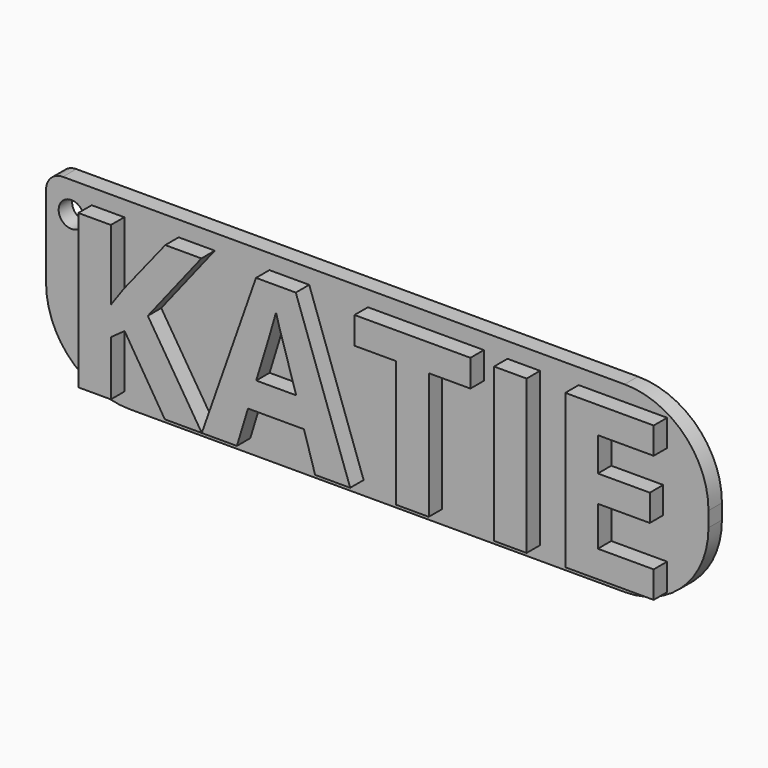
from build123d import *

# Parameters (mm, degrees)
F0_TEXT_SIZE = 32.5522437278
F2_DEPTH     = 5.08
F1_W         = 100.2589799464
F1_H         = 27.6808142662
F3_DEPTH     = 2.54
F4_R         = 12.7
F5_R         = 2.54
F6_R         = 1.9295612823
F7_DEPTH     = 2.54


# Not quite as in the source:
# - Text() gives the source's letters only with a copy of the font that has no kerning and outlines rounded to 1/6400 em; it was checked with that copy


with BuildPart() as f2:
    # F0 (on Front) → F2 (new body)
    with BuildSketch(Plane.XZ):
        with Locations((-40.1719734073, 18.204908818)):
            Text('KATIE', F0_TEXT_SIZE, font='Open Sans', font_style=FontStyle.BOLD, text_align=(TextAlign.LEFT, TextAlign.BOTTOM))
    extrude(amount=F2_DEPTH)


with BuildPart() as f3:
    # F1 (on face) → F3 (new body)
    with BuildSketch(Plane.XZ):
        with Locations((5.9745330364, 29.9661830068)):
            Rectangle(F1_W, F1_H)
    extrude(amount=F3_DEPTH)

    # F4
    f4_edges = [f3.edges().sort_by_distance(p)[0] for p in [
        (-44.154957, -1.27, 16.125776),
        (56.104023, -1.27, 43.80659),
        (56.104023, -1.27, 16.125776),
    ]]
    fillet(f4_edges, radius=F4_R)

    # F5
    f5_edges = [f3.edges().sort_by_distance(p)[0] for p in [
        (-44.154957, -1.27, 43.80659),
    ]]
    fillet(f5_edges, radius=F5_R)

    # F6 (on Front) → F7 (cut)
    with BuildSketch(Plane.XZ):
        with Locations((-40.3213470029, 39.2110511751)):
            Circle(F6_R)
    extrude(amount=F7_DEPTH, mode=Mode.SUBTRACT)


solid = Compound([f2.part, f3.part])
